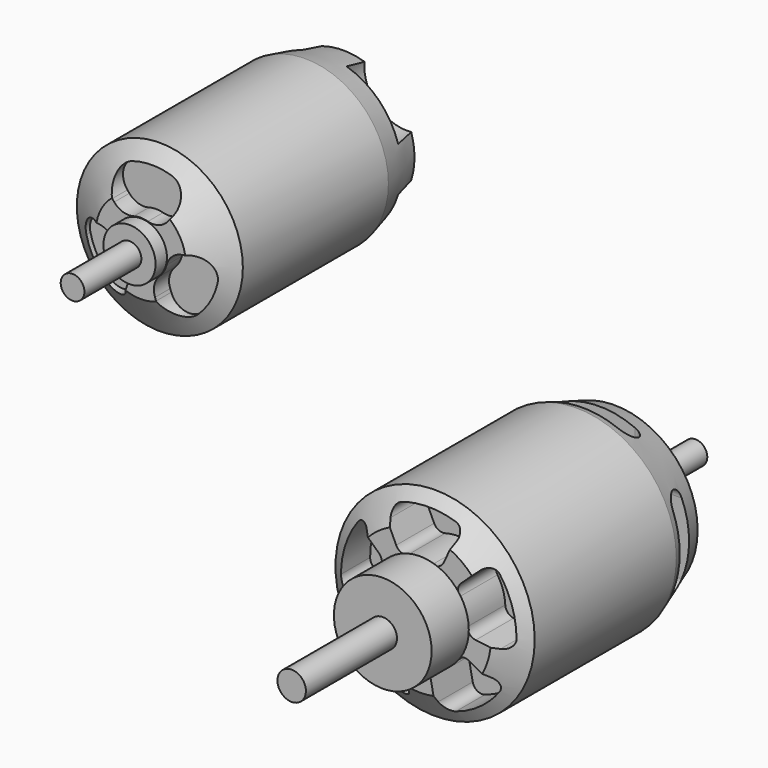
from build123d import *

# Parameters (mm, degrees)
F0_R           = 21
F1_DEPTH       = 51.3
F3_SIZE2       = 4
F3_SIZE        = 6
F4_SIZE2       = 3.5
F4_SIZE        = 10
F5_DEPTH       = 10
F6_R           = 4
F6_R_2         = 1.5
F7_DEPTH       = 8
F9_R           = 2.5
F10_DEPTH      = 21.3
F12_DEPTH      = 21.0010001
F12_DEPTH_BACK = 21.0010001
F14_DEPTH      = 25
F14_DEPTH_BACK = 25
F8_R           = 5.5
F15_DEPTH      = 7
F15_DEPTH_BACK = 50
F16_R          = 1
F17_DEPTH      = 3
F18_R          = 10.3
F18_R_2        = 5.5
F19_DEPTH      = 7
F20_R          = 10.3
F21_DEPTH      = 2.8
F22_R          = 3
F23_DEPTH      = 24
F24_R          = 17.5
F25_DEPTH      = 53.35
F26_SIZE2      = 5
F26_SIZE       = 8
F27_SIZE2      = 2.5
F27_SIZE       = 10
F29_DEPTH      = 4
F30_R          = 5.5
F31_DEPTH      = 3
F32_R          = 2.5
F33_DEPTH      = 15
F34_R          = 2.5
F35_DEPTH      = 6.3
F36_R          = 1.5
F36_R_2        = 9
F37_DEPTH      = 5


with BuildPart() as f1:
    # F0 (on Front) → F1 (new body)
    with BuildSketch(Plane.XZ):
        Circle(F0_R)
    extrude(amount=F1_DEPTH)

    # F3
    f3_edges = [f1.edges().sort_by_distance(p)[0] for p in [
        (-21, -51.3, 0),
    ]]
    f3_side = f1.faces().sort_by_distance((0, -51.3, 0))[0]
    chamfer(f3_edges, length=F3_SIZE, length2=F3_SIZE2, reference=f3_side)

    # F4
    f4_edges = [f1.edges().sort_by_distance(p)[0] for p in [
        (-21, 0, 0),
    ]]
    f4_side = f1.faces().sort_by_distance((-21, -23.65, 0))[0]
    chamfer(f4_edges, length=F4_SIZE, length2=F4_SIZE2, reference=f4_side)

    # F2 (on face) → F5 (cut)
    with BuildSketch(Plane.XZ.offset(51.3)):
        with BuildLine():
            ThreePointArc((-11.743964443, -1.4419775174), (-10.5201730609, -0.8156918585), (-9.9897526082, 0.4525956549))
            ThreePointArc((-9.9897526082, 0.4525956549), (-9.510565163, 3.0901699437), (-8.3479086808, 5.5056716808))
            ThreePointArc((-8.3479086808, 5.5056716808), (-8.0315471452, 6.8435111525), (-8.6534936969, 8.0695134201))
            Line((-8.6534936969, 8.0695134201), (-11.978359113, 11.1700005801))
            ThreePointArc((-11.978359113, 11.1700005801), (-13.5333882451, 11.6981489269), (-14.9596110857, 10.883934774))
            ThreePointArc((-14.9596110857, 10.883934774), (-17.5945455515, 5.7168143959), (-18.4999959446, -0.0122494217))
            ThreePointArc((-18.4999959446, -0.0122494217), (-17.8247405001, -1.5092752606), (-16.2562576962, -1.9960174632))
            Line((-16.2562576962, -1.9960174632), (-11.743964443, -1.4419775174))
        make_face()
        with BuildLine():
            ThreePointArc((-5.0004867085, 10.7235783523), (-4.0266813169, 9.7532164957), (-2.6565592787, 9.6406790632))
            ThreePointArc((-2.6565592787, 9.6406790632), (0, 10), (2.6565592787, 9.6406790632))
            ThreePointArc((2.6565592787, 9.6406790632), (4.0266813169, 9.7532164957), (5.0004867085, 10.7235783523))
            Line((5.0004867085, 10.7235783523), (6.9217853081, 14.8438164954))
            ThreePointArc((6.9217853081, 14.8438164954), (6.9435538063, 16.4859438992), (5.7284630351, 17.5907564151))
            ThreePointArc((5.7284630351, 17.5907564151), (0, 18.5), (-5.7284630351, 17.5907564151))
            ThreePointArc((-5.7284630351, 17.5907564151), (-6.9435538063, 16.4859438992), (-6.9217853081, 14.8438164954))
            Line((-6.9217853081, 14.8438164954), (-5.0004867085, 10.7235783523))
        make_face()
        with BuildLine():
            ThreePointArc((8.6534936969, 8.0695134201), (8.0315471452, 6.8435111525), (8.3479086808, 5.5056716808))
            ThreePointArc((8.3479086808, 5.5056716808), (9.510565163, 3.0901699437), (9.9897526082, 0.4525956549))
            ThreePointArc((9.9897526082, 0.4525956549), (10.5201730609, -0.8156918585), (11.743964443, -1.4419775174))
            Line((11.743964443, -1.4419775174), (16.2562576962, -1.9960174632))
            ThreePointArc((16.2562576962, -1.9960174632), (17.8247405001, -1.5092752606), (18.4999959446, -0.0122494217))
            ThreePointArc((18.4999959446, -0.0122494217), (17.5945455515, 5.7168143959), (14.9596110857, 10.883934774))
            ThreePointArc((14.9596110857, 10.883934774), (13.5333882451, 11.6981489269), (11.978359113, 11.1700005801))
            Line((11.978359113, 11.1700005801), (8.6534936969, 8.0695134201))
        make_face()
        with BuildLine():
            ThreePointArc((10.3486399346, -5.736344786), (8.9904504349, -5.5236940011), (7.8158505784, -6.2379868336))
            ThreePointArc((7.8158505784, -6.2379868336), (5.8778525229, -8.0901699437), (3.5174473724, -9.3609595653))
            ThreePointArc((3.5174473724, -9.3609595653), (2.4751432023, -10.2573417886), (2.25768248, -11.6147694691))
            Line((2.25768248, -11.6147694691), (3.1251344781, -16.0774231298))
            ThreePointArc((3.1251344781, -16.0774231298), (4.0727416634, -17.4187273086), (5.7051632505, -17.5983269741))
            ThreePointArc((5.7051632505, -17.5983269741), (10.8740271674, -14.9668143959), (14.9740111445, -10.8641147934))
            ThreePointArc((14.9740111445, -10.8641147934), (15.3076477247, -9.2560902569), (14.3248183694, -7.9403764826))
            Line((14.3248183694, -7.9403764826), (10.3486399346, -5.736344786))
        make_face()
        with BuildLine():
            ThreePointArc((-2.25768248, -11.6147694691), (-2.4751432023, -10.2573417886), (-3.5174473724, -9.3609595653))
            ThreePointArc((-3.5174473724, -9.3609595653), (-5.8778525229, -8.0901699437), (-7.8158505784, -6.2379868336))
            ThreePointArc((-7.8158505784, -6.2379868336), (-8.9904504349, -5.5236940011), (-10.3486399346, -5.736344786))
            Line((-10.3486399346, -5.736344786), (-14.3248183694, -7.9403764826))
            ThreePointArc((-14.3248183694, -7.9403764826), (-15.3076477247, -9.2560902569), (-14.9740111445, -10.8641147934))
            ThreePointArc((-14.9740111445, -10.8641147934), (-10.8740271674, -14.9668143959), (-5.7051632505, -17.5983269741))
            ThreePointArc((-5.7051632505, -17.5983269741), (-4.0727416634, -17.4187273086), (-3.1251344781, -16.0774231298))
            Line((-3.1251344781, -16.0774231298), (-2.25768248, -11.6147694691))
        make_face()
    extrude(amount=-F5_DEPTH, mode=Mode.SUBTRACT)

    # F6 (on face) → F7 (cut)
    with BuildSketch(Plane(origin=(0, 0, 0), x_dir=(-1, 0, 0), z_dir=(0, 1, 0))):
        with Locations((0, 12.5)):
            Circle(F6_R)
        with Locations((8.8388347648, 8.8388347648)):
            Circle(F6_R_2)
        with Locations((-12.5, 0)):
            Circle(F6_R)
        with Locations((-8.8388347648, 8.8388347648)):
            Circle(F6_R_2)
        with Locations((0, -12.5)):
            Circle(F6_R)
        with Locations((-8.8388347648, -8.8388347648)):
            Circle(F6_R_2)
        with Locations((12.5, 0)):
            Circle(F6_R)
        with Locations((8.8388347648, -8.8388347648)):
            Circle(F6_R_2)
    extrude(amount=-F7_DEPTH, mode=Mode.SUBTRACT)

    # F9 (on face) → F10 (join)
    with BuildSketch(Plane(origin=(0, 0, 0), x_dir=(-1, 0, 0), z_dir=(0, 1, 0))):
        Circle(F9_R)
    extrude(amount=F10_DEPTH)

    # F11 (on Right) → F12 (cut, two sides)
    with BuildSketch(Plane.YZ) as f12_sk:
        with BuildLine():
            Line((-4, -7.5), (-4, 7.5))
            ThreePointArc((-4, 7.5), (-6.2, 9.7), (-8.4, 7.5))
            Line((-8.4, 7.5), (-8.4, -7.5))
            ThreePointArc((-8.4, -7.5), (-6.2, -9.7), (-4, -7.5))
        make_face()
    extrude(amount=F12_DEPTH, mode=Mode.SUBTRACT)
    extrude(f12_sk.sketch, amount=-F12_DEPTH_BACK, mode=Mode.SUBTRACT)

    # F13 (on Top) → F14 (cut, two sides)
    with BuildSketch(Plane.XY) as f14_sk:
        with BuildLine():
            Line((7.499998901, -4), (-7.500001099, -4))
            ThreePointArc((-7.500001099, -4), (-9.700001099, -6.2), (-7.500001099, -8.4))
            Line((-7.500001099, -8.4), (7.499998901, -8.4))
            ThreePointArc((7.499998901, -8.4), (9.699998901, -6.2), (7.499998901, -4))
        make_face()
    extrude(amount=-F14_DEPTH, mode=Mode.SUBTRACT)
    extrude(f14_sk.sketch, amount=F14_DEPTH_BACK, mode=Mode.SUBTRACT)

    # F8 (on face) → F15 (join, two sides)
    with BuildSketch(Plane.XZ.offset(51.3)) as f15_sk:
        Circle(F8_R)
    extrude(amount=F15_DEPTH)
    extrude(f15_sk.sketch, amount=-F15_DEPTH_BACK)

    # F16 (on face) → F17 (cut)
    with BuildSketch(Plane.XZ.offset(51.3)):
        with Locations((0, -8)):
            Circle(F16_R)
        with Locations((6.9282032303, 4)):
            Circle(F16_R)
        with Locations((-6.9282032303, 4)):
            Circle(F16_R)
    extrude(amount=-F17_DEPTH, mode=Mode.SUBTRACT)


with BuildPart() as f19:
    # F18 (on face) → F19 (new body)
    with BuildSketch(Plane.XZ.offset(51.3)):
        Circle(F18_R)
        Circle(F18_R_2, mode=Mode.SUBTRACT)
    extrude(amount=F19_DEPTH)

    # F20 (on face) → F21 (join)
    with BuildSketch(Plane.XZ.offset(58.3)):
        Circle(F20_R)
    extrude(amount=F21_DEPTH)

    # F22 (on face) → F23 (join)
    with BuildSketch(Plane.XZ.offset(61.1)):
        Circle(F22_R)
    extrude(amount=F23_DEPTH)


with BuildPart() as f25:
    # F24 (on Front) → F25 (new body)
    with BuildSketch(Plane.XZ):
        with Locations((-57.1910180151, 49.7522577643)):
            Circle(F24_R)
    extrude(amount=F25_DEPTH)

    # F26
    f26_edges = [f25.edges().sort_by_distance(p)[0] for p in [
        (-74.691018, -53.35, 49.752258),
    ]]
    f26_side = f25.faces().sort_by_distance((-57.191018, -53.35, 49.752258))[0]
    chamfer(f26_edges, length=F26_SIZE, length2=F26_SIZE2, reference=f26_side)

    # F27
    f27_edges = [f25.edges().sort_by_distance(p)[0] for p in [
        (-74.691018, 0, 49.752258),
    ]]
    f27_side = f25.faces().sort_by_distance((-74.691018, -24.175, 49.752258))[0]
    chamfer(f27_edges, length=F27_SIZE, length2=F27_SIZE2, reference=f27_side)

    # F28 (on face) → F29 (cut)
    with BuildSketch(Plane.XZ.offset(53.35)):
        with BuildLine():
            ThreePointArc((-53.0603845132, 63.3382014884), (-57.1910180151, 63.9522577643), (-61.3216515171, 63.3382014884))
            ThreePointArc((-61.3216515171, 63.3382014884), (-63.9924904824, 60.6502072604), (-63.2222705566, 56.9400246485))
            Line((-63.2222705566, 56.9400246485), (-62.8006060031, 56.4375044019))
            ThreePointArc((-62.8006060031, 56.4375044019), (-60.9267381685, 55.1898641615), (-58.6758406408, 55.1518227255))
            ThreePointArc((-58.6758406408, 55.1518227255), (-57.1910180151, 55.3522577643), (-55.7061953895, 55.1518227255))
            ThreePointArc((-55.7061953895, 55.1518227255), (-53.4552978618, 55.1898641615), (-51.5814300272, 56.4375044019))
            Line((-51.5814300272, 56.4375044019), (-51.1597654737, 56.9400246485))
            ThreePointArc((-51.1597654737, 56.9400246485), (-50.3895455479, 60.6502072604), (-53.0603845132, 63.3382014884))
        make_face()
        with BuildLine():
            ThreePointArc((-60.1758174399, 41.5515887432), (-60.0322632141, 43.7982260115), (-61.1247671281, 45.7665811698))
            ThreePointArc((-61.1247671281, 45.7665811698), (-62.0407602763, 46.9522577643), (-62.6095897538, 48.3383693977))
            ThreePointArc((-62.6095897538, 48.3383693977), (-63.7679833675, 50.26868312), (-65.7854054278, 51.2676801479))
            Line((-65.7854054278, 51.2676801479), (-66.431433004, 51.3815922398))
            ThreePointArc((-66.431433004, 51.3815922398), (-70.0296553616, 50.1935309561), (-71.0221071655, 46.5365194487))
            ThreePointArc((-71.0221071655, 46.5365194487), (-69.4885787489, 42.6522577643), (-66.8914736636, 39.3820523559))
            ThreePointArc((-66.8914736636, 39.3820523559), (-63.2281828943, 38.4130350765), (-60.4001804626, 40.9351564047))
            Line((-60.4001804626, 40.9351564047), (-60.1758174399, 41.5515887432))
        make_face()
        with BuildLine():
            ThreePointArc((-48.5966306024, 51.2676801479), (-50.6140526628, 50.26868312), (-51.7724462765, 48.3383693977))
            ThreePointArc((-51.7724462765, 48.3383693977), (-52.341275754, 46.9522577643), (-53.2572689022, 45.7665811698))
            ThreePointArc((-53.2572689022, 45.7665811698), (-54.3497728161, 43.7982260115), (-54.2062185904, 41.5515887432))
            Line((-54.2062185904, 41.5515887432), (-53.9818555677, 40.9351564047))
            ThreePointArc((-53.9818555677, 40.9351564047), (-51.153853136, 38.4130350765), (-47.4905623667, 39.3820523559))
            ThreePointArc((-47.4905623667, 39.3820523559), (-44.8934572814, 42.6522577643), (-43.3599288648, 46.5365194487))
            ThreePointArc((-43.3599288648, 46.5365194487), (-44.3523806687, 50.1935309561), (-47.9506030263, 51.3815922398))
            Line((-47.9506030263, 51.3815922398), (-48.5966306024, 51.2676801479))
        make_face()
    extrude(amount=-F29_DEPTH, mode=Mode.SUBTRACT)

    # F30 (on face) → F31 (join)
    with BuildSketch(Plane.XZ.offset(53.35)):
        with Locations((-57.1910180151, 49.7522577643)):
            Circle(F30_R)
    extrude(amount=F31_DEPTH)

    # F32 (on face) → F33 (join)
    with BuildSketch(Plane.XZ.offset(56.35)):
        with Locations((-57.1910180151, 49.7522577643)):
            Circle(F32_R)
    extrude(amount=F33_DEPTH)

    # F34 (on face) → F35 (join)
    with BuildSketch(Plane(origin=(0, 0, 0), x_dir=(-1, 0, 0), z_dir=(0, 1, 0))):
        with Locations((57.1910180151, 49.7522577643)):
            Circle(F34_R)
    extrude(amount=F35_DEPTH)

    # F36 (on face) → F37 (cut)
    with BuildSketch(Plane(origin=(0, 0, 0), x_dir=(-1, 0, 0), z_dir=(0, 1, 0))):
        with Locations((57.1910180151, 62.2522577643)):
            Circle(F36_R)
        with Locations((70.6260468577, 63.1872866069)):
            Circle(F36_R_2)
        with Locations((43.7559891726, 63.1872866069)):
            Circle(F36_R_2)
        with Locations((44.6910180151, 49.7522577643)):
            Circle(F36_R)
        with Locations((43.7559891726, 36.3172289218)):
            Circle(F36_R_2)
        with Locations((57.1910180151, 37.2522577643)):
            Circle(F36_R)
        with Locations((70.6260468577, 36.3172289218)):
            Circle(F36_R_2)
        with Locations((69.6910180151, 49.7522577643)):
            Circle(F36_R)
    extrude(amount=-F37_DEPTH, mode=Mode.SUBTRACT)


solid = Compound([f1.part, f19.part, f25.part])
